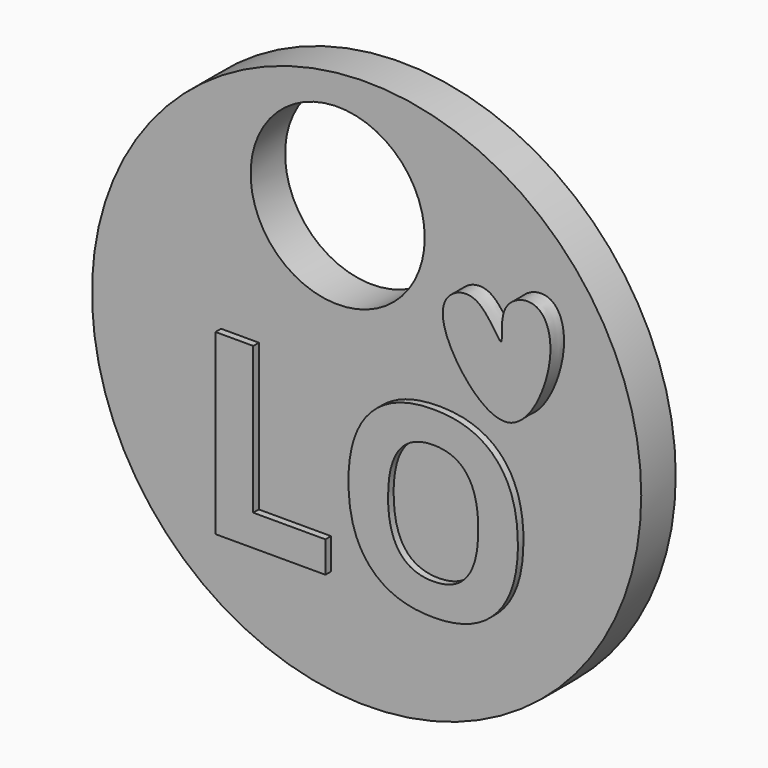
from build123d import *

# Parameters (mm, degrees)
F0_R         = 13.7
F1_DEPTH     = 2.15
F2_R         = 4.3422904904
F3_DEPTH     = 2.15
F4_TEXT_SIZE = 12.436372021
F5_DEPTH     = 2.5
F7_DEPTH     = 3


# Not quite as in the source:
# - Text() gives the source's letters only with a copy of the font that has no kerning and outlines rounded to 1/6400 em; it was checked with that copy


with BuildPart() as f1:
    # F0 (on Front) → F1 (new body)
    with BuildSketch(Plane.XZ):
        with Locations((-33.5059948266, 26.1404532939)):
            Circle(F0_R)
    extrude(amount=F1_DEPTH)

    # F2 (on Front) → F3 (cut, through all)
    with BuildSketch(Plane.XZ):
        with Locations((-34.9502153695, 33.9392609894)):
            Circle(F2_R)
    extrude(amount=F3_DEPTH, mode=Mode.SUBTRACT)

    # F4 (on Front) → F5 (join)
    with BuildSketch(Plane.XZ):
        with Locations((-41.8824926019, 17.763953656)):
            Text('LO', F4_TEXT_SIZE, font='Open Sans', font_style=FontStyle.BOLD, text_align=(TextAlign.LEFT, TextAlign.BOTTOM))
    extrude(amount=F5_DEPTH)

    # F6 (on Front) → F7 (join)
    with BuildSketch(Plane.XZ):
        with BuildLine():
            add(Edge.make_bspline(
                [(-25.704825297, 27.7607310563), (-26.7048568834, 27.5365150069), (-28.8440980288, 29.7992038441), (-29.3204889431, 32.3432125258), (-27.1656331588, 33.1604944328), (-25.8261442788, 30.2365536915), (-26.3543453739, 32.9580692552), (-24.2186014729, 33.8113569588), (-23.1378167763, 31.3965297953), (-24.6187000401, 28.0042500787), (-25.704825297, 27.7607310563)],
                knots=[0, 0, 0, 0, 0.1575373723, 0.284292953, 0.3881083224, 0.5011439863, 0.6018373242, 0.7078956095, 0.8289000854, 1, 1, 1, 1], degree=3))
        make_face()
    extrude(amount=F7_DEPTH)


solid = f1.part
